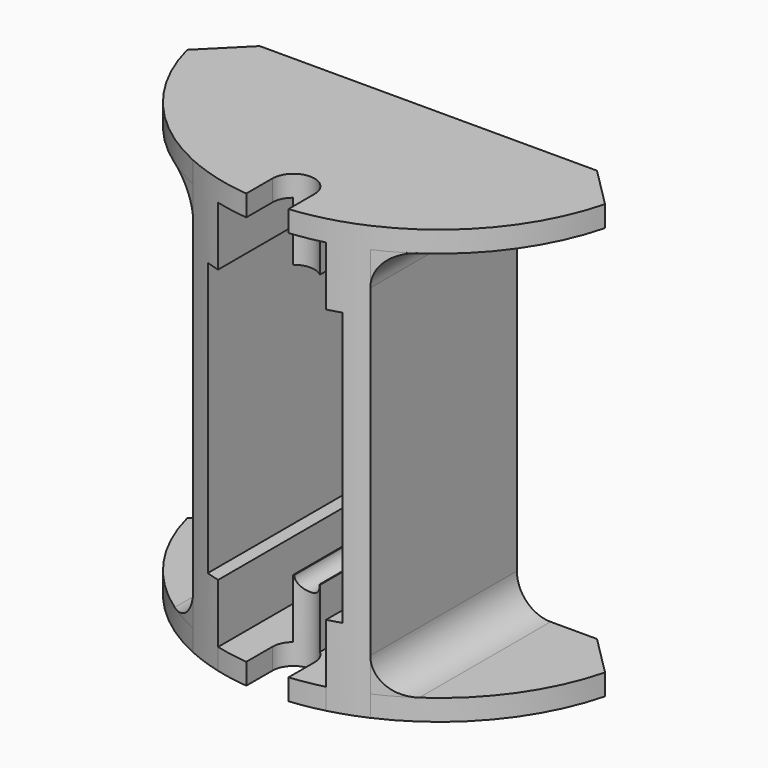
from build123d import *

# Parameters (mm, degrees)
F0_W          = 26.67
F0_H          = 58.928
F0_R          = 1.5875
F1_DEPTH      = 3.175
F2_W          = 4.064
F2_H          = 8.89
F3_DEPTH      = 38.1
F5_DEPTH      = 101.6
F7_DEPTH      = 3.175
F9_DEPTH      = 3.175
F11_DEPTH     = 127
F12_T4_DEPTH  = 40.3062822545
F12_S5_R      = 32.5
F12_T6_DEPTH  = 22
F12_T10_DEPTH = 40.3062822545
F12_S11_R     = 32.5
F12_T12_DEPTH = 22
F12_T16_DEPTH = 40.3062822545
F12_S17_R     = 32.5
F12_T18_DEPTH = 22
F12_T22_DEPTH = 40.3062822545
F12_S23_R     = 32.5
F12_T24_DEPTH = 22


# Not quite as in the source:
# - a fillet or chamfer that OpenCascade refuses, or shapes differently, is made with other operations: its cross-section is extruded or revolved along the edge and cut away or added
# - after a boolean that leaves OpenCascade's solid faulty, fix() repairs it


with BuildPart() as f1:
    # F0 (on Front) → F1 (new body)
    with BuildSketch(Plane.XZ):
        with Locations((-10.16, 20.574)):
            Rectangle(F0_W, F0_H)
        with Locations((-15.24, -3.81)):
            Circle(F0_R, mode=Mode.SUBTRACT)
        with BuildLine():
            Line((0, 41.148), (0, 0))
            Line((0, 0), (-8.255, 0))
            ThreePointArc((-8.255, 0), (-10.16, -1.905), (-12.065, 0))
            Line((-12.065, 0), (-20.32, 0))
            Line((-20.32, 0), (-20.32, 41.148))
            Line((-20.32, 41.148), (0, 41.148))
        make_face(mode=Mode.SUBTRACT)
        with Locations((-5.08, -3.81)):
            Circle(F0_R, mode=Mode.SUBTRACT)
        with Locations((-15.24, 44.958)):
            Circle(F0_R, mode=Mode.SUBTRACT)
        with Locations((-5.08, 44.958)):
            Circle(F0_R, mode=Mode.SUBTRACT)
    extrude(amount=F1_DEPTH)

    # F2 (on face) → F3 (join)
    with BuildSketch(Plane.XZ.offset(3.175)):
        Polygon((0, 0), (-2.032, 0), (-2.032, -8.89), (3.175, -8.89), (3.175, 50.038), (-2.032, 50.038), (-2.032, 41.148), (0, 41.148), align=None)
        with BuildLine():
            Line((-8.128, -8.89), (-8.128, 0))
            Line((-8.128, 0), (-8.255, 0))
            ThreePointArc((-8.255, 0), (-10.16, -1.905), (-12.065, 0))
            Line((-12.065, 0), (-12.192, 0))
            Line((-12.192, 0), (-12.192, -8.89))
            Line((-12.192, -8.89), (-8.128, -8.89))
        make_face()
        Polygon((-23.495, -8.89), (-18.288, -8.89), (-18.288, 0), (-20.32, 0), (-20.32, 41.148), (-18.288, 41.148), (-18.288, 50.038), (-23.495, 50.038), align=None)
        with Locations((-10.16, 45.593)):
            Rectangle(F2_W, F2_H)
    extrude(amount=F3_DEPTH)

    # F4 (on face) → F5 (intersect)
    with BuildSketch(Plane.XY.offset(50.038)):
        with BuildLine():
            Line((-23.495, 0), (-23.495, -27.6062822545))
            ThreePointArc((-23.495, -27.6062822545), (-20.9303918657, -28.6314743475), (-18.288, -29.4352149387))
            Line((-18.288, -29.4352149387), (-18.288, -3.175))
            Line((-18.288, -3.175), (-12.192, -3.175))
            Line((-12.192, -3.175), (-12.192, -30.4044143518))
            ThreePointArc((-12.192, -30.4044143518), (-10.16, -30.468), (-8.128, -30.4044143518))
            Line((-8.128, -30.4044143518), (-8.128, -3.175))
            Line((-8.128, -3.175), (-2.032, -3.175))
            Line((-2.032, -3.175), (-2.032, -29.4352149387))
            ThreePointArc((-2.032, -29.4352149387), (0.6103918657, -28.6314743475), (3.175, -27.6062822545))
            Line((3.175, -27.6062822545), (3.175, 0))
            Line((3.175, 0), (-10.16, 0))
            Line((-10.16, 0), (-23.495, 0))
        make_face()
    extrude(amount=-F5_DEPTH, mode=Mode.INTERSECT)

    # F6 (on face) → F7 (join)
    with BuildSketch(Plane(origin=(0, 0, -8.89), x_dir=(1, 0, 0), z_dir=(0, 0, -1))):
        with BuildLine():
            Line((15.24, 0), (21.313116807, 6.073116807))
            ThreePointArc((21.313116807, 6.073116807), (14.6968126777, 18.9057377838), (3.175, 27.6062822545))
            Line((3.175, 27.6062822545), (3.175, 0))
            Line((3.175, 0), (15.24, 0))
        make_face()
        with BuildLine():
            Line((3.175, 0), (3.175, 27.6062822545))
            ThreePointArc((3.175, 27.6062822545), (0.6103918657, 28.6314743475), (-2.032, 29.4352149387))
            Line((-2.032, 29.4352149387), (-2.032, 3.175))
            Line((-2.032, 3.175), (-8.128, 3.175))
            Line((-8.128, 3.175), (-8.128, 30.4044143518))
            ThreePointArc((-8.128, 30.4044143518), (-10.16, 30.468), (-12.192, 30.4044143518))
            Line((-12.192, 30.4044143518), (-12.192, 3.175))
            Line((-12.192, 3.175), (-18.288, 3.175))
            Line((-18.288, 3.175), (-18.288, 29.4352149387))
            ThreePointArc((-18.288, 29.4352149387), (-20.9303918657, 28.6314743475), (-23.495, 27.6062822545))
            Line((-23.495, 27.6062822545), (-23.495, 0))
            Line((-23.495, 0), (-10.16, 0))
            Line((-10.16, 0), (3.175, 0))
        make_face()
        with BuildLine():
            Line((-2.032, 3.175), (-2.032, 29.4352149387))
            ThreePointArc((-2.032, 29.4352149387), (-5.0569384801, 30.0648653162), (-8.128, 30.4044143518))
            Line((-8.128, 30.4044143518), (-8.128, 3.175))
            Line((-8.128, 3.175), (-2.032, 3.175))
        make_face()
        with BuildLine():
            Line((-12.192, 3.175), (-12.192, 30.4044143518))
            ThreePointArc((-12.192, 30.4044143518), (-15.2630615199, 30.0648653162), (-18.288, 29.4352149387))
            Line((-18.288, 29.4352149387), (-18.288, 3.175))
            Line((-18.288, 3.175), (-12.192, 3.175))
        make_face()
        with BuildLine():
            Line((-35.56, 0), (-23.495, 0))
            Line((-23.495, 0), (-23.495, 27.6062822545))
            ThreePointArc((-23.495, 27.6062822545), (-35.0168126777, 18.9057377838), (-41.633116807, 6.073116807))
            Line((-41.633116807, 6.073116807), (-35.56, 0))
        make_face()
    extrude(amount=F7_DEPTH)

    add(f1.part.fix(), mode=Mode.REPLACE)

    # F8 (on face) → F9 (join)
    with BuildSketch(Plane.XY.offset(50.038)):
        with BuildLine():
            Line((-23.495, -27.6062822545), (-23.495, 0))
            Line((-23.495, 0), (-35.56, 0))
            Line((-35.56, 0), (-41.633116807, -6.073116807))
            ThreePointArc((-41.633116807, -6.073116807), (-35.0168126777, -18.9057377838), (-23.495, -27.6062822545))
        make_face()
        with BuildLine():
            Line((15.24, 0), (3.175, 0))
            Line((3.175, 0), (3.175, -27.6062822545))
            ThreePointArc((3.175, -27.6062822545), (14.6968126777, -18.9057377838), (21.313116807, -6.073116807))
            Line((21.313116807, -6.073116807), (15.24, 0))
        make_face()
        with BuildLine():
            Line((-18.288, -3.175), (-18.288, -29.4352149387))
            ThreePointArc((-18.288, -29.4352149387), (-15.2630615199, -30.0648653162), (-12.192, -30.4044143518))
            Line((-12.192, -30.4044143518), (-12.192, -3.175))
            Line((-12.192, -3.175), (-18.288, -3.175))
        make_face()
        with BuildLine():
            ThreePointArc((-8.128, -30.4044143518), (-5.0569384801, -30.0648653162), (-2.032, -29.4352149387))
            Line((-2.032, -29.4352149387), (-2.032, -3.175))
            Line((-2.032, -3.175), (-8.128, -3.175))
            Line((-8.128, -3.175), (-8.128, -30.4044143518))
        make_face()
        with BuildLine():
            Line((3.175, -27.6062822545), (3.175, 0))
            Line((3.175, 0), (-23.495, 0))
            Line((-23.495, 0), (-23.495, -27.6062822545))
            ThreePointArc((-23.495, -27.6062822545), (-20.9303918657, -28.6314743475), (-18.288, -29.4352149387))
            Line((-18.288, -29.4352149387), (-18.288, -3.175))
            Line((-18.288, -3.175), (-12.192, -3.175))
            Line((-12.192, -3.175), (-12.192, -30.4044143518))
            ThreePointArc((-12.192, -30.4044143518), (-10.16, -30.468), (-8.128, -30.4044143518))
            Line((-8.128, -30.4044143518), (-8.128, -3.175))
            Line((-8.128, -3.175), (-2.032, -3.175))
            Line((-2.032, -3.175), (-2.032, -29.4352149387))
            ThreePointArc((-2.032, -29.4352149387), (0.6103918657, -28.6314743475), (3.175, -27.6062822545))
        make_face()
    extrude(amount=F9_DEPTH)

    # F10 (on face) → F11 (cut)
    with BuildSketch(Plane(origin=(0, 0, -12.065), x_dir=(1, 0, 0), z_dir=(0, 0, -1))):
        with BuildLine():
            Line((-13.335, 30.312541657), (-13.335, 25.4))
            ThreePointArc((-13.335, 25.4), (-10.16, 22.225), (-6.985, 25.4))
            Line((-6.985, 25.4), (-6.985, 30.312541657))
            ThreePointArc((-6.985, 30.312541657), (-10.16, 30.468), (-13.335, 30.312541657))
        make_face()
    extrude(amount=-F11_DEPTH, mode=Mode.SUBTRACT)

    # F12: fillet of radius 5.08 on 4 edges, made by hand


with BuildPart() as f12_tool2:
    # F12_s3 → F12_t4 (new body)
    with BuildSketch(Plane.XZ.offset(40.3062822545)):
        with BuildLine():
            ThreePointArc((-23.495, -3.81), (-24.9828975516, -7.4021024484), (-28.575, -8.89))
            Line((-28.575, -8.89), (-23.495, -8.89))
            Line((-23.495, -8.89), (-23.495, -3.81))
        make_face()
    extrude(amount=-F12_T4_DEPTH)

    # F12_s5 → F12_t6 (intersect, symmetric)
    with BuildSketch(Plane.XY.offset(-6.4)):
        with Locations((-10.16, 2.032)):
            Circle(F12_S5_R)
    extrude(amount=F12_T6_DEPTH, both=True, mode=Mode.INTERSECT)


with BuildPart() as f1_1:
    add(f1.part)

    # F12_t1: union F12_tool2
    add(f12_tool2.part)


with BuildPart() as f12_tool8:
    # F12_s9 → F12_t10 (new body)
    with BuildSketch(Plane.XZ):
        with BuildLine():
            ThreePointArc((-28.575, 50.038), (-24.9828975516, 48.5501024484), (-23.495, 44.958))
            Line((-23.495, 44.958), (-23.495, 50.038))
            Line((-23.495, 50.038), (-28.575, 50.038))
        make_face()
    extrude(amount=F12_T10_DEPTH)

    # F12_s11 → F12_t12 (intersect, symmetric)
    with BuildSketch(Plane.XY.offset(47.5)):
        with Locations((-10.16, 2.032)):
            Circle(F12_S11_R)
    extrude(amount=F12_T12_DEPTH, both=True, mode=Mode.INTERSECT)


with BuildPart() as f1_2:
    add(f1_1.part)

    # F12_t7: union F12_tool8
    add(f12_tool8.part)


with BuildPart() as f12_tool14:
    # F12_s15 → F12_t16 (new body)
    with BuildSketch(Plane.XZ):
        with BuildLine():
            ThreePointArc((3.175, 44.958), (4.6628975516, 48.5501024484), (8.255, 50.038))
            Line((8.255, 50.038), (3.175, 50.038))
            Line((3.175, 50.038), (3.175, 44.958))
        make_face()
    extrude(amount=F12_T16_DEPTH)

    # F12_s17 → F12_t18 (intersect, symmetric)
    with BuildSketch(Plane.XY.offset(47.5)):
        with Locations((-10.16, 2.032)):
            Circle(F12_S17_R)
    extrude(amount=F12_T18_DEPTH, both=True, mode=Mode.INTERSECT)


with BuildPart() as f1_3:
    add(f1_2.part)

    # F12_t13: union F12_tool14
    add(f12_tool14.part)


with BuildPart() as f12_tool20:
    # F12_s21 → F12_t22 (new body)
    with BuildSketch(Plane.XZ.offset(40.3062822545)):
        with BuildLine():
            ThreePointArc((8.255, -8.89), (4.6628975516, -7.4021024484), (3.175, -3.81))
            Line((3.175, -3.81), (3.175, -8.89))
            Line((3.175, -8.89), (8.255, -8.89))
        make_face()
    extrude(amount=-F12_T22_DEPTH)

    # F12_s23 → F12_t24 (intersect, symmetric)
    with BuildSketch(Plane.XY.offset(-6.4)):
        with Locations((-10.16, 2.032)):
            Circle(F12_S23_R)
    extrude(amount=F12_T24_DEPTH, both=True, mode=Mode.INTERSECT)


with BuildPart() as f1_4:
    add(f1_3.part)

    # F12_t19: union F12_tool20
    add(f12_tool20.part)


solid = f1_4.part
